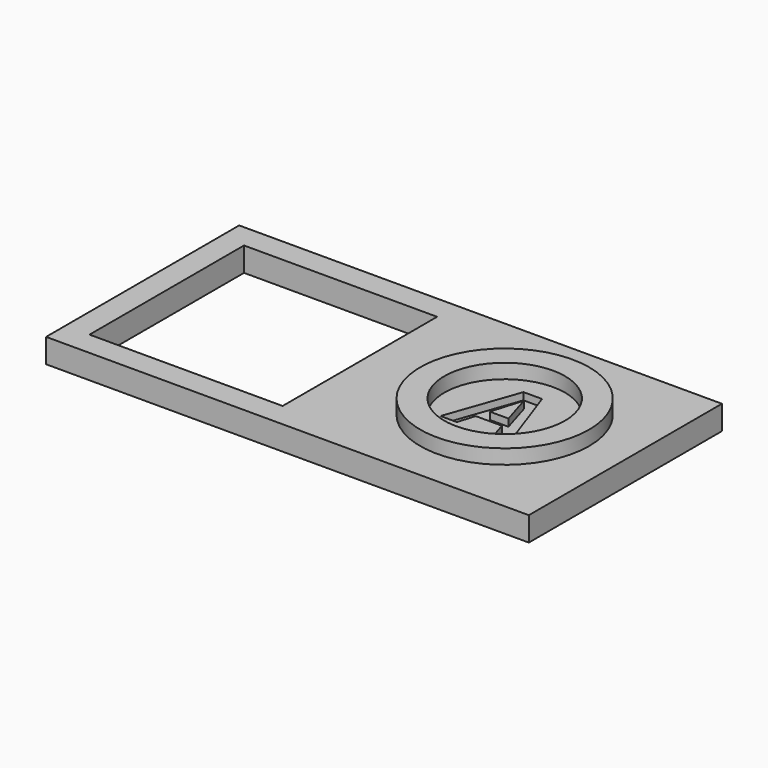
from build123d import *

# Parameters (mm, degrees)
F0_W         = 100
F0_H         = 50
F0_W_2       = 40
F0_H_2       = 40
F1_DEPTH     = 5
F2_R         = 17.5
F2_R_2       = 12.5
F3_DEPTH     = 3
F4_TEXT_SIZE = 20.8333333333
F5_DEPTH     = 1.5


# Not quite as in the source:
# - Text() gives the source's letters only with a copy of the font that has no kerning and outlines rounded to 1/6400 em; it was checked with that copy


with BuildPart() as f1:
    # F0 (on Top) → F1 (new body)
    with BuildSketch(Plane.XY):
        Rectangle(F0_W, F0_H)
        with Locations((-25, 0)):
            Rectangle(F0_W_2, F0_H_2, mode=Mode.SUBTRACT)
    extrude(amount=F1_DEPTH)

    # F2 (on face) → F3 (join)
    with BuildSketch(Plane.XY.offset(5)):
        with Locations((25, 0)):
            Circle(F2_R)
        with Locations((25, 0)):
            Circle(F2_R_2, mode=Mode.SUBTRACT)
    extrude(amount=F3_DEPTH)

    # F4 (on face) → F5 (cut)
    with BuildSketch(Plane.XY.offset(5)):
        with Locations((17.1370442708, -6.807129782)):
            Text('A', F4_TEXT_SIZE, font='Open Sans', font_style=FontStyle.BOLD, text_align=(TextAlign.LEFT, TextAlign.BOTTOM))
    extrude(amount=-F5_DEPTH, mode=Mode.SUBTRACT)


solid = f1.part
